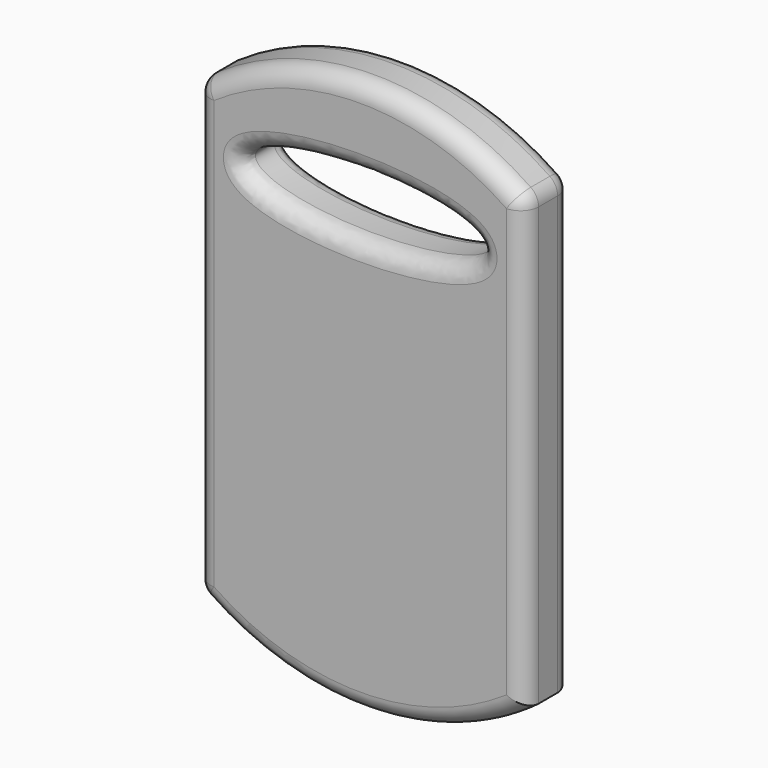
from build123d import *

# Parameters (mm, degrees)
F1_DEPTH = 5
F2_R     = 1.5


with BuildPart() as f1:
    # F0 (on Front) → F1 (new body)
    with BuildSketch(Plane.XZ):
        with BuildLine():
            Line((13.7920752168, 9.5829919425), (13.7920752168, 47.1181124449))
            ThreePointArc((13.7920752168, 47.1181124449), (0, 51.6409505709), (-13.7920752168, 47.1181124449))
            Line((-13.7920752168, 47.1181124449), (-13.7920752168, 9.5829919425))
            ThreePointArc((-13.7920752168, 9.5829919425), (0, 5.0601538166), (13.7920752168, 9.5829919425))
        make_face()
        with BuildLine():
            add(Edge.make_bspline(
                [(-10, 42.3880703747), (-10, 38.0579433558), (5, 40.2230068653), (20, 42.3880703747), (5, 44.5531338842), (-10, 46.7181973936), (-10, 42.3880703747)],
                knots=[0, 0, 0, 2.0943951024, 2.0943951024, 4.1887902048, 4.1887902048, 6.2831853072, 6.2831853072, 6.2831853072], degree=2, weights=[1, 0.5, 1, 0.5, 1, 0.5, 1]))
        make_face(mode=Mode.SUBTRACT)
    extrude(amount=F1_DEPTH)

    # F2
    f2_edges = [f1.edges().sort_by_distance(p)[0] for p in [
        (0, -5, 51.640951),
        (-13.792075, -5, 28.350552),
        (0, -5, 5.060154),
        (13.792075, -5, 28.350552),
        (-13.792075, -2.5, 47.118112),
        (-13.792075, -2.5, 9.582992),
        (0, 0, 51.640951),
        (13.792075, -2.5, 47.118112),
        (13.792075, 0, 28.350552),
        (0, 0, 5.060154),
        (10, 0, 42.387712),
        (10, -5, 42.387712),
    ]]
    fillet(f2_edges, radius=F2_R)


solid = f1.part
